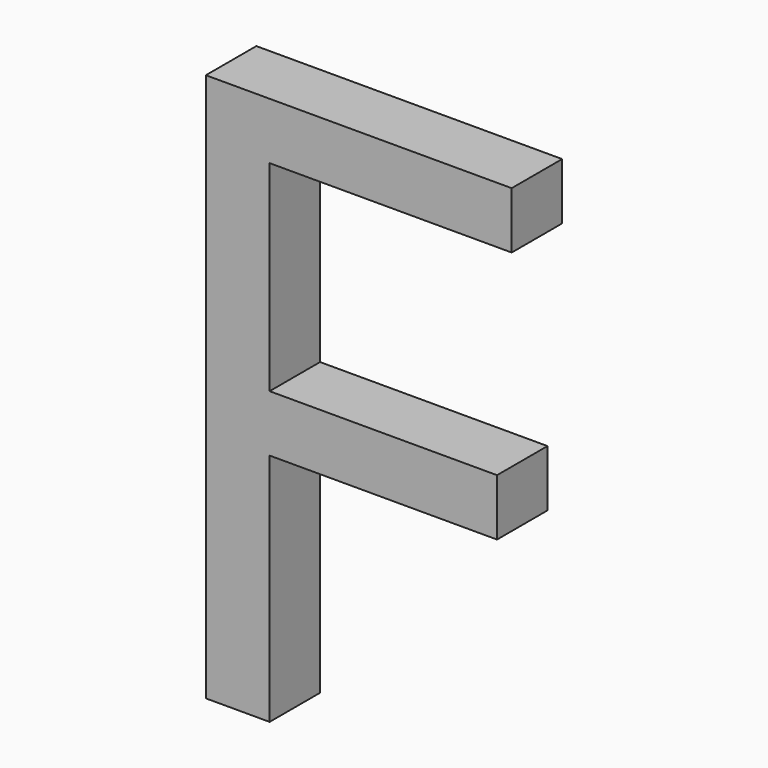
from build123d import *

# Parameters (mm, degrees)
F0_TEXT_SIZE = 92.8338280775
F1_DEPTH     = 7.62


# Not quite as in the source:
# - Text() gives the source's letters only with a copy of the font that has no kerning and outlines rounded to 1/6400 em; it was checked with that copy


with BuildPart() as f1:
    # F0 (on Front) → F1 (new body)
    with BuildSketch(Plane.XZ):
        with Locations((-30.7749509811, -27.4845454842)):
            Text('F', F0_TEXT_SIZE, font='Open Sans', text_align=(TextAlign.LEFT, TextAlign.BOTTOM))
    extrude(amount=F1_DEPTH)


solid = f1.part
